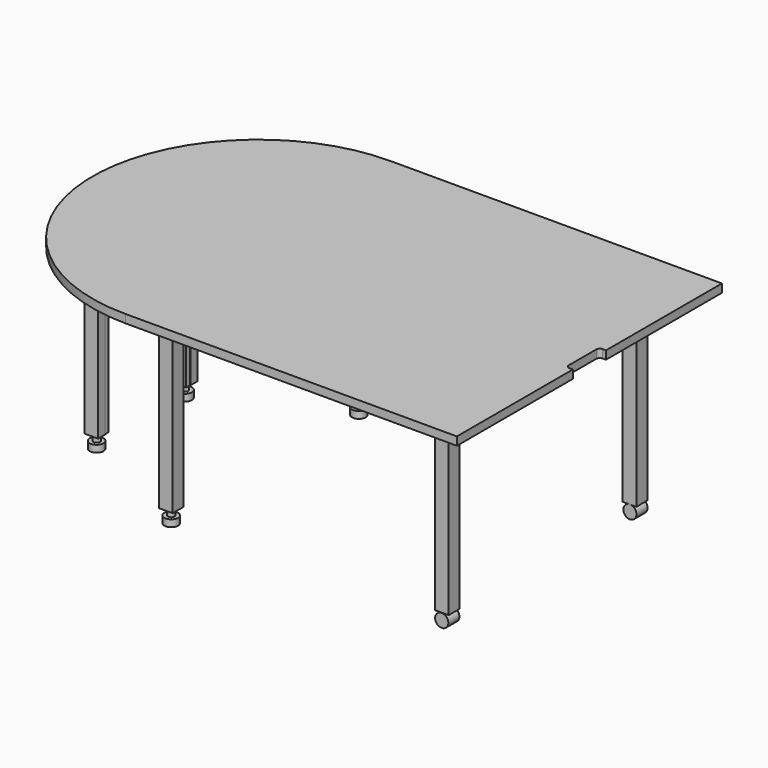
from build123d import *

# Parameters (mm, degrees)
F1_DEPTH  = 30.48
F3_DEPTH  = 50.8
F5_DEPTH  = 609.6
F4_W      = 50.8
F4_H      = 50.8
F6_DEPTH  = 609.6
F7_R      = 24.2659285134
F8_DEPTH  = 50.8
F10_R     = 12.2300412489
F11_DEPTH = 25.4
F10_R_2   = 12.192
F12_R     = 25.4
F12_R_2   = 12.2300412489
F13_DEPTH = 25.4
F15_DEPTH = 30.48


# Not quite as in the source:
# - a feature names something its author has since deleted; it is built from what else it names


with BuildPart() as f1:
    # F0 (on Top) → F1 (new body)
    with BuildSketch(Plane.XY):
        with BuildLine():
            Line((1219.2, 0), (0, 0))
            ThreePointArc((0, 0), (431.0522938113, -178.5477061887), (609.6, -609.6))
            ThreePointArc((609.6, -609.6), (431.0522938113, -1040.6522938113), (0, -1219.2))
            Line((0, -1219.2), (1219.2, -1219.2))
            Line((1219.2, -1219.2), (1219.2, -685.8))
            Line((1219.2, -685.8), (1206.5, -685.8))
            ThreePointArc((1206.5, -685.8), (1197.5197438789, -682.0802561211), (1193.8, -673.1))
            Line((1193.8, -673.1), (1193.8, -609.6))
            Line((1193.8, -609.6), (1193.8, -546.1))
            ThreePointArc((1193.8, -546.1), (1197.5197438789, -537.1197438789), (1206.5, -533.4))
            Line((1206.5, -533.4), (1219.2, -533.4))
            Line((1219.2, -533.4), (1219.2, 0))
        make_face()
        with BuildLine():
            Line((0, -1219.2), (0, 0))
            ThreePointArc((0, 0), (-609.6, -609.6), (0, -1219.2))
        make_face()
        with BuildLine():
            ThreePointArc((609.6, -609.6), (431.0522938113, -178.5477061887), (0, 0))
            Line((0, 0), (0, -1219.2))
            ThreePointArc((0, -1219.2), (431.0522938113, -1040.6522938113), (609.6, -609.6))
        make_face()
    extrude(amount=-F1_DEPTH)


with BuildPart() as f3:
    # F2 (on face) → F3 (new body)
    with BuildSketch(Plane(origin=(0, 0, -30.48), x_dir=(1, 0, 0), z_dir=(0, 0, -1))):
        Polygon((1066.8, 152.4), (1066.8, 609.6), (1066.8, 1066.8), (0, 1066.8), (-457.2, 838.2), (-457.2, 609.6), (-457.2, 381), (0, 152.4), align=None)
        Polygon((-407.8729450703, 805.2982634406), (13.5305280485, 1016), (1016, 1016), (1016, 609.6), (1016, 203.2), (13.5305280485, 203.2), (-407.8729450703, 413.9017365594), (-407.8729450703, 609.6), align=None, mode=Mode.SUBTRACT)
    extrude(amount=F3_DEPTH)

    # F4 (on face) → F5 (join)
    with BuildSketch(Plane(origin=(0, 0, -81.28), x_dir=(1, 0, 0), z_dir=(0, 0, -1))):
        Polygon((50.8, 1016), (50.8, 1066.8), (0, 1066.8), (0, 1016), (13.5305280485, 1016), align=None)
        Polygon((50.8, 152.4), (50.8, 203.2), (13.5305280485, 203.2), (0, 203.2), (0, 152.4), align=None)
        Polygon((-406.4, 381), (-406.4, 413.1652640242), (-407.8729450703, 413.9017365594), (-407.8729450703, 431.8), (-457.2, 431.8), (-457.2, 381), align=None)
        Polygon((-406.4, 838.2), (-457.2, 838.2), (-457.2, 787.4), (-407.8729450703, 787.4), (-407.8729450703, 805.2982634406), (-406.4, 806.0347359758), align=None)
    extrude(amount=F5_DEPTH)

    # F4 (on face) → F6 (join)
    with BuildSketch(Plane(origin=(0, 0, -81.28), x_dir=(1, 0, 0), z_dir=(0, 0, -1))):
        with Locations((1041.4, 1041.4)):
            Rectangle(F4_W, F4_H)
        with Locations((1041.4, 177.8)):
            Rectangle(F4_W, F4_H)
    extrude(amount=F6_DEPTH)


with BuildPart() as f8:
    # F7 (on face) → F8 (new body)
    with BuildSketch(Plane.XZ.offset(1066.8)):
        with Locations((1041.4, -716.2297964096)):
            Circle(F7_R)
    extrude(amount=-F8_DEPTH)


with BuildPart() as f9_1:
    # F9: copy of F8
    add(f8.part.moved(Location((0, 865.632, 0))))


with BuildPart() as f11:
    # F10 (on face) → F11 (new body)
    with BuildSketch(Plane(origin=(0, 0, -690.88), x_dir=(1, 0, 0), z_dir=(0, 0, -1))):
        with Locations((25.4, 1041.4)):
            Circle(F10_R)
    extrude(amount=F11_DEPTH)

    # F12 (on face) → F13 (join)
    with BuildSketch(Plane(origin=(0, 0, -716.28), x_dir=(1, 0, 0), z_dir=(0, 0, -1))):
        with Locations((25.4, 1041.4)):
            Circle(F12_R)
        with Locations((25.4, 1041.4)):
            Circle(F12_R_2, mode=Mode.SUBTRACT)
        with Locations((25.4, 1041.4)):
            Circle(F12_R_2)
    extrude(amount=F13_DEPTH)


with BuildPart() as f11b:
    # F10 (on face) → F11, piece 2 (new body)
    with BuildSketch(Plane(origin=(0, 0, -690.88), x_dir=(1, 0, 0), z_dir=(0, 0, -1))):
        with Locations((-431.8, 812.8)):
            Circle(F10_R_2)
    extrude(amount=F11_DEPTH)

    # F12 (on face) → F13, piece 4 (join)
    with BuildSketch(Plane(origin=(0, 0, -716.28), x_dir=(1, 0, 0), z_dir=(0, 0, -1))):
        with Locations((-431.8, 812.8)):
            Circle(F12_R)
    extrude(amount=F13_DEPTH)


with BuildPart() as f11c:
    # F10 (on face) → F11, piece 3 (new body)
    with BuildSketch(Plane(origin=(0, 0, -690.88), x_dir=(1, 0, 0), z_dir=(0, 0, -1))):
        with Locations((-431.8, 406.4)):
            Circle(F10_R_2)
    extrude(amount=F11_DEPTH)

    # F12 (on face) → F13, piece 2 (join)
    with BuildSketch(Plane(origin=(0, 0, -716.28), x_dir=(1, 0, 0), z_dir=(0, 0, -1))):
        with Locations((-431.8, 406.4)):
            Circle(F12_R)
    extrude(amount=F13_DEPTH)


with BuildPart() as f11d:
    # F10 (on face) → F11, piece 4 (new body)
    with BuildSketch(Plane(origin=(0, 0, -690.88), x_dir=(1, 0, 0), z_dir=(0, 0, -1))):
        with Locations((25.4, 177.8)):
            Circle(F10_R)
    extrude(amount=F11_DEPTH)

    # F12 (on face) → F13, piece 3 (join)
    with BuildSketch(Plane(origin=(0, 0, -716.28), x_dir=(1, 0, 0), z_dir=(0, 0, -1))):
        with Locations((25.4, 177.8)):
            Circle(F12_R)
    extrude(amount=F13_DEPTH)


with BuildPart() as f15:
    # F14 (on face) → F15 (new body)
    with BuildSketch(Plane(origin=(0, 0, -30.48), x_dir=(1, 0, 0), z_dir=(0, 0, -1))):
        with BuildLine():
            ThreePointArc((876.1052652473, 678.833677063), (874.3197881855, 683.1442000011), (870.0092652473, 684.929677063))
            Line((870.0092652473, 684.929677063), (617.6992004356, 684.929677063))
            ThreePointArc((617.6992004356, 684.929677063), (613.3886774975, 683.1442000011), (611.6032004356, 678.833677063))
            Line((611.6032004356, 678.833677063), (611.6032004356, 677.4499876404))
            ThreePointArc((611.6032004356, 677.4499876404), (613.3886774975, 673.1394647023), (617.6992004356, 671.3539876404))
            Line((617.6992004356, 671.3539876404), (870.0092652473, 671.3539876404))
            ThreePointArc((870.0092652473, 671.3539876404), (874.3197881855, 673.1394647023), (876.1052652473, 677.4499876404))
            Line((876.1052652473, 677.4499876404), (876.1052652473, 678.833677063))
        make_face()
    extrude(amount=F15_DEPTH)


with BuildPart() as f15b:
    # F14 (on face) → F15, piece 2 (new body)
    with BuildSketch(Plane(origin=(0, 0, -30.48), x_dir=(1, 0, 0), z_dir=(0, 0, -1))):
        with BuildLine():
            Line((882.3782937622, 552.6862859154), (798.9836199188, 552.6862859154))
            ThreePointArc((798.9836199188, 552.6862859154), (788.2073125735, 548.2225932607), (783.7436199188, 537.4462859154))
            Line((783.7436199188, 537.4462859154), (783.7436199188, 395.8324355984))
            ThreePointArc((783.7436199188, 395.8324355984), (788.2073125735, 385.0561282531), (798.9836199188, 380.5924355984))
            Line((798.9836199188, 380.5924355984), (882.3782937622, 380.5924355984))
            ThreePointArc((882.3782937622, 380.5924355984), (893.1546011075, 385.0561282531), (897.6182937622, 395.8324355984))
            Line((897.6182937622, 395.8324355984), (897.6182937622, 537.4462859154))
            ThreePointArc((897.6182937622, 537.4462859154), (893.1546011075, 548.2225932607), (882.3782937622, 552.6862859154))
        make_face()
    extrude(amount=F15_DEPTH)


solid = Compound([f1.part, f3.part, f8.part, f9_1.part, f11.part, f11b.part, f11c.part, f11d.part, f15.part, f15b.part])
